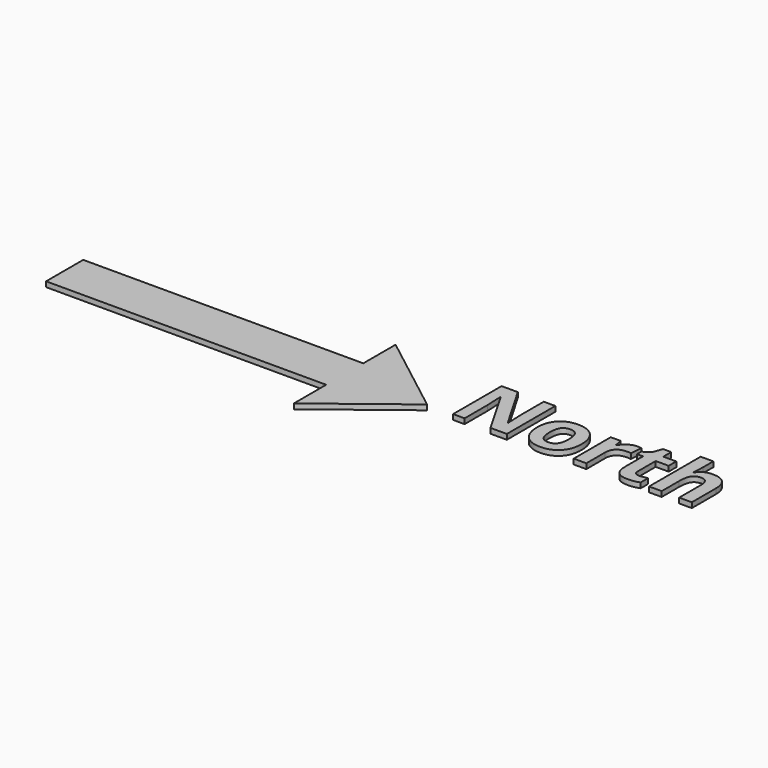
from build123d import *

# Parameters (mm, degrees)
F1_DEPTH     = 25
F0_TEXT_SIZE = 409.8290189484
F3_DEPTH     = 25


# Not quite as in the source:
# - Text() gives the source's letters only with a copy of the font that has no kerning and outlines rounded to 1/6400 em; it was checked with that copy


with BuildPart() as f1:
    # F0 (on Top) → F1 (new body)
    with BuildSketch(Plane.XY):
        Polygon((-747.5871443748, 112.064242363), (-747.5871443748, 0), (1002.1966695786, 0), (604.6236157417, 306.9731593132), (604.6236157417, 112.064242363), align=None)
    extrude(amount=F1_DEPTH)

    # F2: F1 across plane


with BuildPart() as f1_1:
    add(f1.part)
    add(f1.part.mirror(Plane.XZ))


with BuildPart() as f3:
    # F0 (on Top) → F3 (new body)
    with BuildSketch(Plane.XY):
        with Locations((1091.0751542937, 0)):
            Text('North', F0_TEXT_SIZE, font='Open Sans', font_style=FontStyle.BOLD, text_align=(TextAlign.LEFT, TextAlign.BOTTOM))
    extrude(amount=F3_DEPTH)


solid = Compound([f1_1.part, f3.part])
